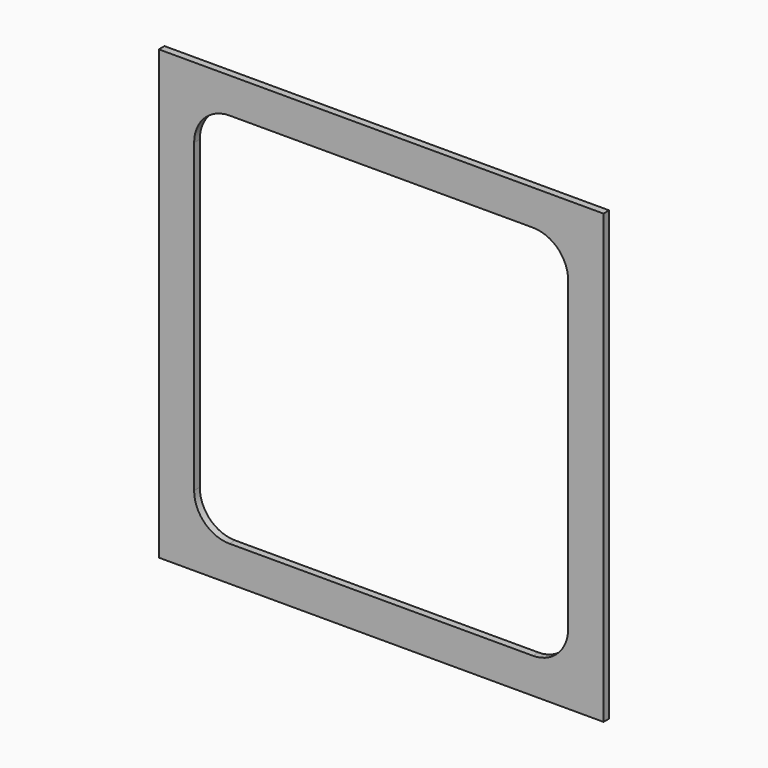
from build123d import *

# Parameters (mm, degrees)
F0_W     = 630
F0_H     = 634
F1_DEPTH = 10


# Not quite as in the source:
# - a feature names something its author has since deleted; it is built from what else it names


with BuildPart() as f1:
    # F0 (on Front) → F1 (new body)
    with BuildSketch(Plane.XZ):
        with Locations((-26.3475316763, 87.0849853243)):
            Rectangle(F0_W, F0_H)
        with BuildLine():
            ThreePointArc((-291.3475316763, 304.0849853243), (-276.7028707356, 339.4403243836), (-241.3475316763, 354.0849853243))
            Line((-241.3475316763, 354.0849853243), (188.6524683237, 354.0849853243))
            ThreePointArc((188.6524683237, 354.0849853243), (224.007807383, 339.4403243836), (238.6524683237, 304.0849853243))
            Line((238.6524683237, 304.0849853243), (238.6524683237, -129.9150146759))
            ThreePointArc((238.6524683237, -129.9150146759), (224.007807383, -165.2703537352), (188.6524683237, -179.9150146759))
            Line((188.6524683237, -179.9150146759), (-241.3475316763, -179.9150146759))
            ThreePointArc((-241.3475316763, -179.9150146759), (-276.7028707356, -165.2703537352), (-291.3475316763, -129.9150146759))
            Line((-291.3475316763, -129.9150146759), (-291.3475316763, 304.0849853243))
        make_face(mode=Mode.SUBTRACT)
    extrude(amount=F1_DEPTH)


solid = f1.part
